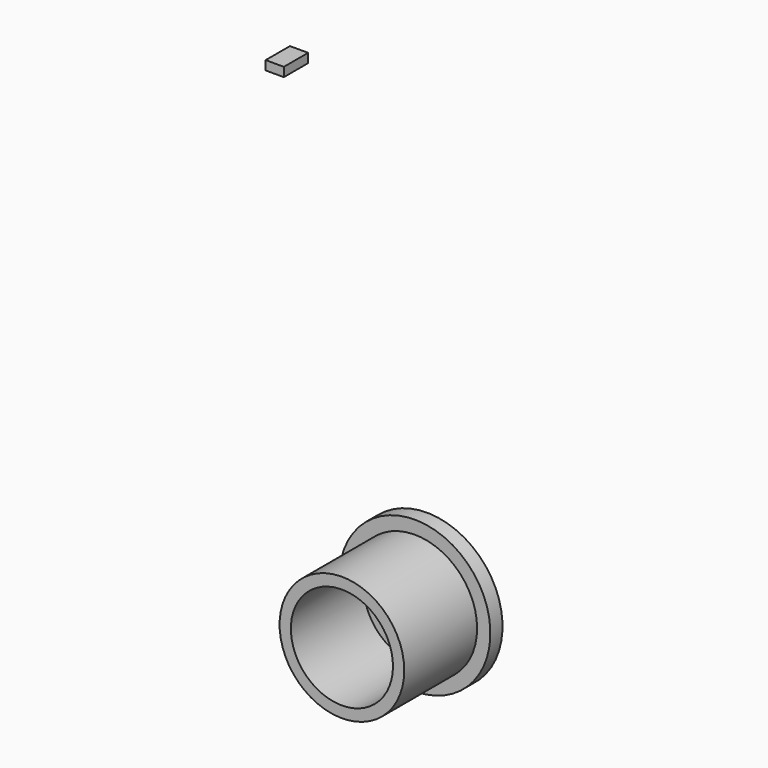
from build123d import *

# Parameters (mm, degrees)
F0_W     = 30
F0_H     = 50
F1_DEPTH = 15
F2_R     = 102.6493082789
F2_R_2   = 84.1005190764
F3_DEPTH = 150
F4_R     = 124.4985615198
F4_R_2   = 102.6493082789
F4_R_3   = 84.1005190764
F5_DEPTH = 25


with BuildPart() as f1:
    # F0 (on Top) → F1 (new body)
    with BuildSketch(Plane.XY):
        with Locations((-1573.3778619766, 386.8347048759)):
            Rectangle(F0_W, F0_H)
    extrude(amount=F1_DEPTH)


with BuildPart() as f3:
    # F2 (on Front) → F3 (new body)
    with BuildSketch(Plane.XZ):
        with Locations((-1053.2720088959, -454.607874155)):
            Circle(F2_R)
        with Locations((-1053.2720088959, -454.607874155)):
            Circle(F2_R_2, mode=Mode.SUBTRACT)
    extrude(amount=F3_DEPTH)

    # F4 (on face) → F5 (join)
    with BuildSketch(Plane(origin=(0, 0, 0), x_dir=(-1, 0, 0), z_dir=(0, 1, 0))):
        with Locations((1053.2720088959, -454.607874155)):
            Circle(F4_R)
        with Locations((1053.2720088959, -454.607874155)):
            Circle(F4_R_2, mode=Mode.SUBTRACT)
        with Locations((1053.2720088959, -454.607874155)):
            Circle(F4_R_2)
        with Locations((1053.2720088959, -454.607874155)):
            Circle(F4_R_3, mode=Mode.SUBTRACT)
        with Locations((1053.2720088959, -454.607874155)):
            Circle(F4_R_3)
    extrude(amount=F5_DEPTH)


solid = Compound([f1.part, f3.part])
